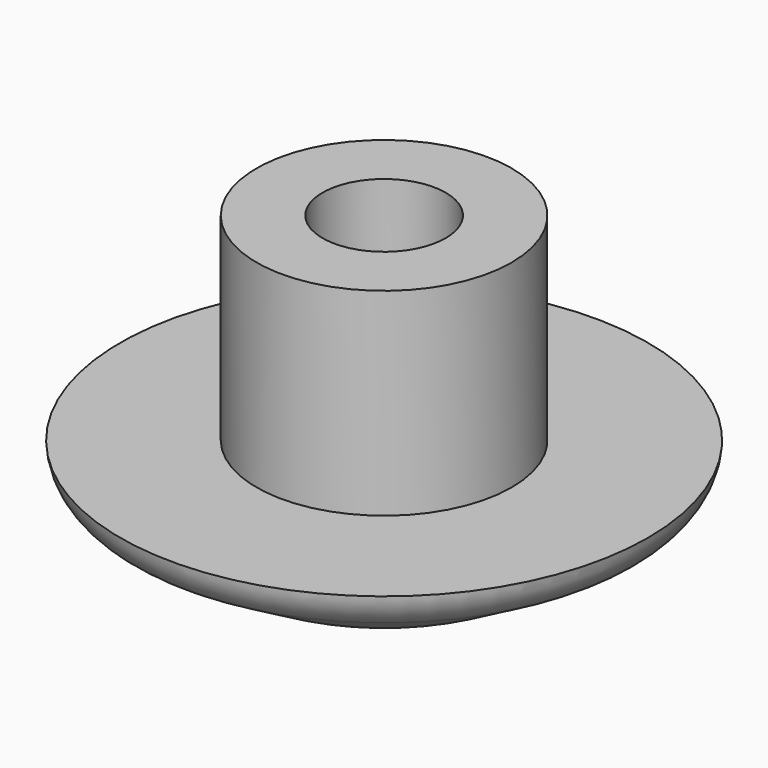
from build123d import *

# Parameters (mm, degrees)
F0_R     = 6
F1_DEPTH = 2
F2_SIZE2 = 2.5980762114
F2_SIZE  = 1.5
F4_R     = 2.9
F4_R_2   = 1.4
F5_DEPTH = 4.5
F6_R     = 1.2


# Not quite as in the source:
# - a fillet or chamfer that OpenCascade refuses, or shapes differently, is made with other operations: its cross-section is extruded or revolved along the edge and cut away or added


with BuildPart() as f1:
    # F0 (on Top) → F1 (new body)
    with BuildSketch(Plane.XY):
        Circle(F0_R)
    extrude(amount=F1_DEPTH)

    # F2
    f2_edges = [f1.edges().sort_by_distance(p)[0] for p in [
        (-6, 0, 0),
    ]]
    f2_side = f1.faces().sort_by_distance((-6, 0, 1))[0]
    chamfer(f2_edges, length=F2_SIZE, length2=F2_SIZE2, reference=f2_side)

    # F3: fillet of radius 1 on 2 edges, made by hand

    # F3_s1 → F3_t2 (revolve, cut)
    with BuildSketch(Plane.XZ):
        with BuildLine():
            ThreePointArc((3.6339745962, 0.1339745962), (3.3927936413, 0.0340741737), (3.1339745962, 0))
            Line((3.1339745962, 0), (3.4019237886, 0))
            Line((3.4019237886, 0), (3.6339745962, 0.1339745962))
        make_face()
    revolve(axis=Axis((0, 0, 0), (0, 0, 1)), mode=Mode.SUBTRACT)

    # F3_s3 → F3_t4 (revolve, cut)
    with BuildSketch(Plane.XZ):
        with BuildLine():
            ThreePointArc((6, 2), (5.8486778537, 1.5452494356), (5.5031382462, 1.2131367327))
            Line((5.5031382462, 1.2131367327), (6, 1.5))
            Line((6, 1.5), (6, 2))
        make_face()
    revolve(axis=Axis((0, 0, 1.5), (0, 0, 1)), mode=Mode.SUBTRACT)

    # F4 (on face) → F5 (join)
    with BuildSketch(Plane.XY.offset(2)):
        Circle(F4_R)
        Circle(F4_R_2, mode=Mode.SUBTRACT)
    extrude(amount=F5_DEPTH)

    # F6
    f6_edges = [f1.edges().sort_by_distance(p)[0] for p in [
        (-1.4, 0, 2),
    ]]
    fillet(f6_edges, radius=F6_R)


solid = f1.part
